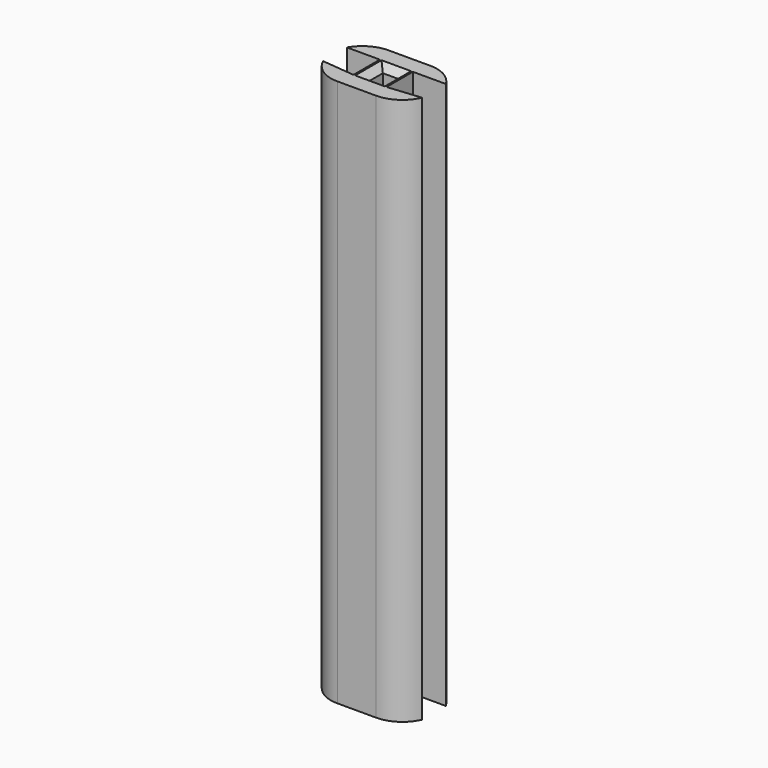
from build123d import *

# Parameters (mm, degrees)
F1_DEPTH    = 83
F2_T1_DEPTH = 104.6506350946
F2_T3_DEPTH = 105.9128784748
F4_W        = 2.5
F4_H        = 3
F5_DEPTH    = 83.001
F6_SIZE     = 1


# Not quite as in the source:
# - a fillet or chamfer that OpenCascade refuses, or shapes differently, is made with other operations: its cross-section is extruded or revolved along the edge and cut away or added


with BuildPart() as f1:
    # F0 (on Top) → F1 (new body)
    with BuildSketch(Plane.XY):
        Polygon((0, -5), (0, 5), (-7.5, 5), (-7.5, 2.5), (-2.5, 2.5), (-2.5, -2.5), (-7.5, -2.5), (-7.5, -5), align=None)
        Polygon((-7.5, -2), (-7.5, -2.5), (-2.5, -2.5), align=None)
    extrude(amount=F1_DEPTH)

    # F2: fillet of radius 5 on 2 edges, made by hand

    # F2_s2 → F2_t1 (cut)
    with BuildSketch(Plane.XY.offset(-10.8253175473)):
        with BuildLine():
            ThreePointArc((-3.1698729811, 5), (-5.6698729811, 4.3301270189), (-7.5, 2.5))
            Line((-7.5, 2.5), (-7.5, 5))
            Line((-7.5, 5), (-3.1698729811, 5))
        make_face()
    extrude(amount=F2_T1_DEPTH, mode=Mode.SUBTRACT)

    # F2_s4 → F2_t3 (cut)
    with BuildSketch(Plane.XY.offset(-11.4564392374)):
        with BuildLine():
            ThreePointArc((-7.5, -2), (-5.6560370926, -4.1833001327), (-2.917424305, -5))
            Line((-2.917424305, -5), (-7.5, -5))
            Line((-7.5, -5), (-7.5, -2))
        make_face()
    extrude(amount=F2_T3_DEPTH, mode=Mode.SUBTRACT)

    # F3: F1 across face


with BuildPart() as f1_1:
    add(f1.part)
    add(f1.part.mirror(Plane(origin=(0, 0, 41.5), x_dir=(0, 1, 0), z_dir=(1, 0, 0))))

    # F4 (on face) → F5 (cut, through all)
    with BuildSketch(Plane.XY.offset(83)):
        Rectangle(F4_W, F4_H)
    extrude(amount=-F5_DEPTH, mode=Mode.SUBTRACT)

    # F6
    f6_edges = [f1_1.edges().sort_by_distance(p)[0] for p in [
        (1.25, 0, 83),
        (0, 1.5, 83),
        (-1.25, 0, 83),
        (0, -1.5, 83),
        (1.25, 0, 0),
        (0, -1.5, 0),
        (-1.25, 0, 0),
        (0, 1.5, 0),
    ]]
    chamfer(f6_edges, length=F6_SIZE)


solid = f1_1.part
